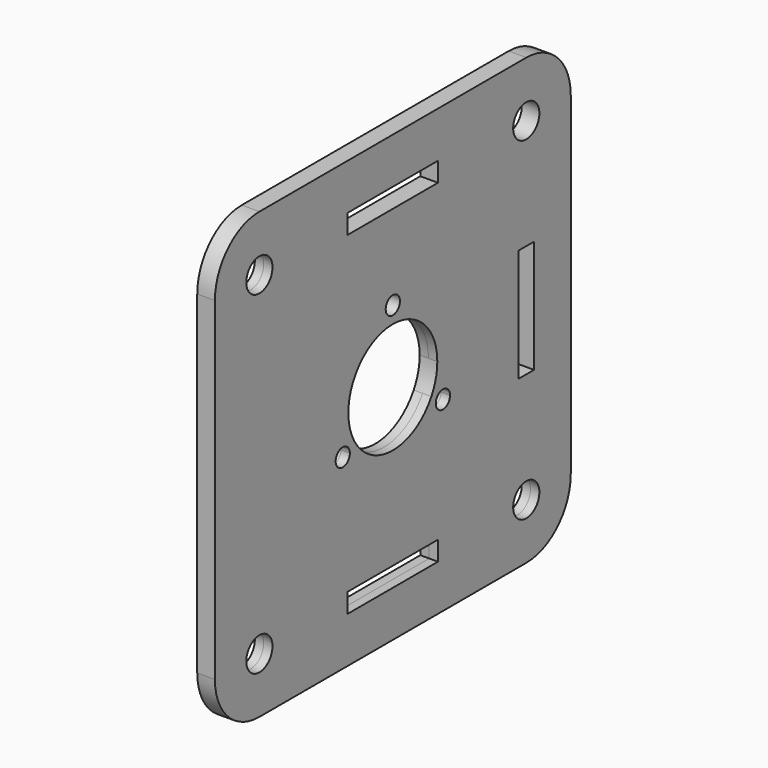
from build123d import *

# Parameters (mm, degrees)
F0_W     = 40
F0_H     = 40
F0_R     = 1.4732
F0_W_2   = 10.15
F0_H_2   = 1.74625
F0_W_3   = 1.74625
F0_H_3   = 10.15
F1_DEPTH = 0.79375
F2_R     = 5


# Not quite as in the source:
# - a length typed as a fraction of an inch, garbled in the dataset ("3 / 203.2 mm" for 3/8 in), is restored


with BuildPart() as f1:
    # F0 (on Right) → F1 (new body, symmetric)
    with BuildSketch(Plane.YZ):
        Rectangle(F0_W, F0_H)
        with Locations((-15, -15)):
            Circle(F0_R, mode=Mode.SUBTRACT)
        with BuildLine():
            ThreePointArc((-4.8291651246, -3.25), (-6.4019057856, -3.4570552361), (-4.9363448016, -2.85))
            ThreePointArc((-4.9363448016, -2.85), (-4.8564244636, -3.0429447639), (-4.8291651246, -3.25))
        make_face(mode=Mode.SUBTRACT)
        with Locations((0, -15)):
            Rectangle(F0_W_2, F0_H_2, mode=Mode.SUBTRACT)
        with Locations((15, -15)):
            Circle(F0_R, mode=Mode.SUBTRACT)
        with BuildLine():
            ThreePointArc((6.4291651246, -3.25), (5.4221098885, -4.022740661), (4.9363448016, -2.85))
            ThreePointArc((4.9363448016, -2.85), (5.8362203607, -2.477259339), (6.4291651246, -3.25))
        make_face(mode=Mode.SUBTRACT)
        with Locations((-15, 15)):
            Circle(F0_R, mode=Mode.SUBTRACT)
        with BuildLine():
            ThreePointArc((0, 5), (3.5355339059, 3.5355339059), (5, 0))
            ThreePointArc((5, 0), (4.8296291314, -1.2940952255), (4.3301270189, -2.5))
            ThreePointArc((4.3301270189, -2.5), (0, -5), (-4.3301270189, -2.5))
            ThreePointArc((-4.3301270189, -2.5), (-4.3301270189, 2.5), (0, 5))
        make_face(mode=Mode.SUBTRACT)
        with BuildLine():
            ThreePointArc((0.8, 6.5), (0.5656854249, 5.9343145751), (0, 5.7))
            ThreePointArc((0, 5.7), (-0.5656854249, 7.0656854249), (0.8, 6.5))
        make_face(mode=Mode.SUBTRACT)
        with Locations((15, 0)):
            Rectangle(F0_W_3, F0_H_3, mode=Mode.SUBTRACT)
        with Locations((0, 15)):
            Rectangle(F0_W_2, F0_H_2, mode=Mode.SUBTRACT)
        with Locations((15, 15)):
            Circle(F0_R, mode=Mode.SUBTRACT)
    extrude(amount=F1_DEPTH, both=True)

    # F2
    f2_edges = [f1.edges().sort_by_distance(p)[0] for p in [
        (0, -20, 20),
        (0, 20, 20),
        (0, -20, -20),
        (0, 20, -20),
    ]]
    fillet(f2_edges, radius=F2_R)


solid = f1.part
